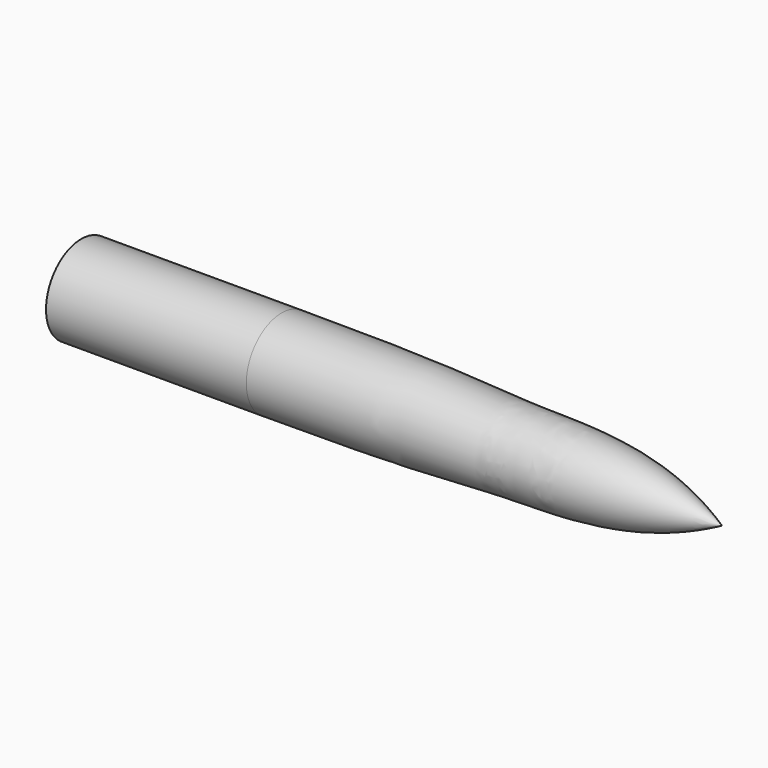
from build123d import *

# Parameters (mm, degrees)
F2_SCALE = 0.5


with BuildPart() as f1:
    # F0 (on Top) → F1 (revolve)
    with BuildSketch(Plane.XY):
        with BuildLine():
            Line((-8.2889255136, 0), (0, 0))
            Line((0, 0), (10.16, 0))
            add(Edge.make_bspline(
                [(-2.521042089, 1.27), (-1.6071708661, 1.27), (1.6580526523, 1.2689667271), (4.6387866527, 1.0284940171), (8.0489429836, 1.1204775711), (10.16, 0)],
                knots=[0, 0, 0, 0, 0.3236529728, 0.6129567303, 1, 1, 1, 1], degree=3))
            Line((-2.521042089, 1.27), (-8.2889255136, 1.27))
            Line((-8.2889255136, 1.27), (-8.2889255136, 0))
        make_face()
    revolve(axis=Axis((5.08, 0, 0), (1, 0, 0)))


with BuildPart() as f1_1:
    # F2: moved
    add(f1.part.scale(F2_SCALE))


solid = f1_1.part
